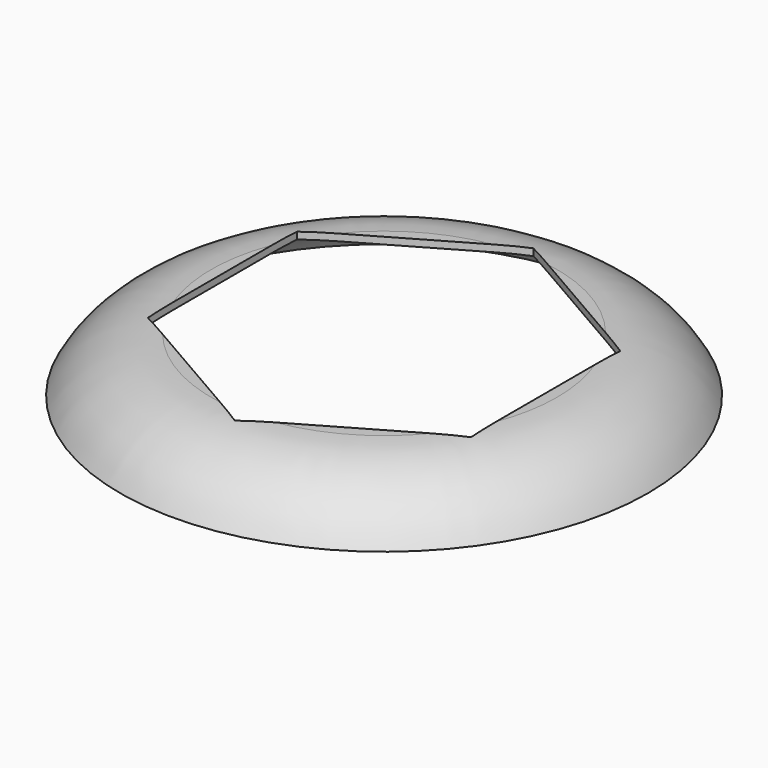
from build123d import *

# Parameters (mm, degrees)
F0_R     = 38.5
F1_DEPTH = 8
F4_DEPTH = 8
F5_T     = -1
F7_DEPTH = 25


# Not quite as in the source:
# - a fillet or chamfer that OpenCascade refuses, or shapes differently, is made with other operations: its cross-section is extruded or revolved along the edge and cut away or added


with BuildPart() as f1:
    # F0 (on Top) → F1 (new body)
    with BuildSketch(Plane.XY):
        Circle(F0_R)
    extrude(amount=F1_DEPTH)

    # F3: fillet of radius 15 on 1 edges, made by hand

    # F3_s1 → F3_t2 (revolve, cut)
    with BuildSketch(Plane.XZ):
        with BuildLine():
            ThreePointArc((38.5, 0), (32.979467531, 5.8452325787), (25.2335008386, 8))
            Line((25.2335008386, 8), (25.2335008386, 8.3))
            Line((25.2335008386, 8.3), (38.5, 8.3))
            Line((38.5, 8.3), (38.8, 8))
            ThreePointArc((38.8, 8), (38.8, 4), (38.7653299832, 0.14))
            Line((38.7653299832, 0.14), (38.5, 0))
        make_face()
    revolve(axis=Axis((0, 0, 8), (0, 0, 1)), mode=Mode.SUBTRACT)

    # F2 (on face) → F4 (cut)
    with BuildSketch(Plane.XY.offset(8)):
        Polygon((-0.0532552026, 25.9807075324), (-22.5265803327, 12.9442334078), (-22.47332513, -13.0364741246), (0.0532552026, -25.9807075324), (22.5265803327, -12.9442334078), (22.47332513, 13.0364741246), align=None)
    extrude(amount=-F4_DEPTH, mode=Mode.SUBTRACT)

    # F5
    f5_openings = [f1.faces().sort_by_distance(p)[0] for p in [
        (-37.411056, 0, 0),
    ]]
    offset(amount=F5_T, openings=f5_openings)

    # F6 (on Top) → F7 (cut)
    with BuildSketch(Plane.XY):
        Polygon((-23.56934, 13.6077647936), (-23.56934, -13.6077647936), (0, -27.2155295872), (23.56934, -13.6077647936), (23.56934, 13.6077647936), (0, 27.2155295872), align=None)
    extrude(amount=F7_DEPTH, mode=Mode.SUBTRACT)


solid = f1.part
